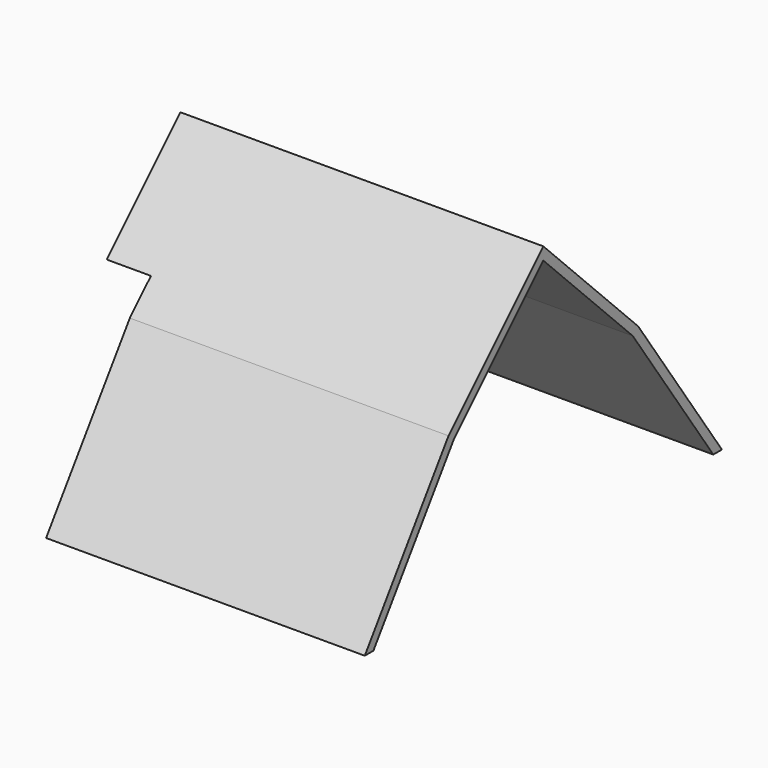
from build123d import *

# Parameters (mm, degrees)
F1_DEPTH = 51
F2_DEPTH = 2
F3_DEPTH = 23
F5_DEPTH = 10


with BuildPart() as f1:
    # F0 (on Right) → F1 (new body)
    with BuildSketch(Plane.YZ):
        Polygon((-106.4311944246, 30.6635548347), (-88.4311944246, 48.6635548347), (-70.4311944246, 30.6635548347), (-63.1831944246, 23.4155548347), (-40.4311944246, -9.4364451653), (-37.9983836671, -9.4364451653), (-61.6478004918, 24.697180939), (-88.4311944246, 51.4919819594), (-115.2145883574, 24.697180939), (-138.8640051821, -9.4364451653), (-136.4311944246, -9.4364451653), (-113.6791944246, 23.4155548347), align=None)
    extrude(amount=F1_DEPTH)

    # F2 (cut): a face of the model
    f2_faces = [f1.faces().sort_by_distance(p)[0] for p in [
        (51, -100.9894629386, 37.2615078041),
    ]]
    extrude(f2_faces, amount=-F2_DEPTH, mode=Mode.SUBTRACT)

    # F3 (add): a face of the model
    f3_faces = [f1.faces().sort_by_distance(p)[0] for p in [
        (0, -100.9894629386, 37.2615078041),
    ]]
    extrude(f3_faces, amount=F3_DEPTH)

    # F4 (on face) → F5 (join)
    with BuildSketch(Plane(origin=(-23, 0, 0), x_dir=(0, -1, 0), z_dir=(-1, 0, 0))):
        Polygon((88.4311944246, 51.4919819594), (67.6116343818, 30.6635548347), (70.4311944246, 30.6635548347), (88.4311944246, 48.6635548347), (106.4311944246, 30.6635548347), (109.2507544675, 30.6635548347), align=None)
    extrude(amount=F5_DEPTH)


solid = f1.part
